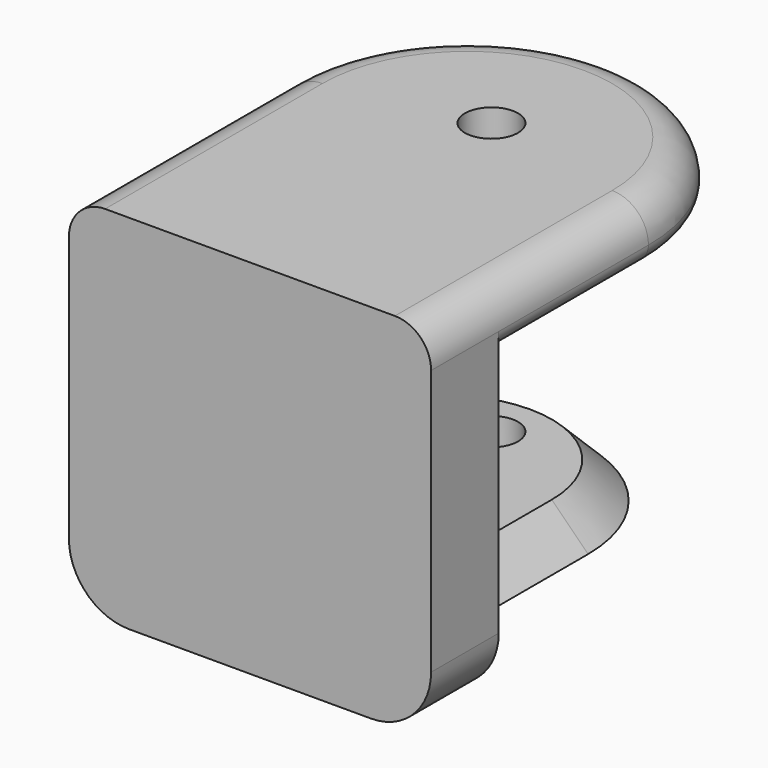
from build123d import *

# Parameters (mm, degrees)
F1_DEPTH  = 7
F3_DEPTH  = 4.5
F4_R      = 3
F5_R      = 1.49999
F7_D      = 4.4
F10_DEPTH = 3
F11_R     = 2.2
F12_DEPTH = 3
F13_SIZE  = 2.99999


# Not quite as in the source:
# - a fillet or chamfer is up to 0.001 mm smaller than in the source, because OpenCascade refuses the exact size


with BuildPart() as f1:
    # F0 (on Front) → F1 (new body)
    with BuildSketch(Plane.XZ):
        with BuildLine():
            Line((15, -10), (15, 15))
            Line((15, 15), (-15, 15))
            Line((-15, 15), (-15, -10))
            ThreePointArc((-15, -10), (-13.5355339059, -13.5355339059), (-10, -15))
            Line((-10, -15), (10, -15))
            ThreePointArc((10, -15), (13.5355339059, -13.5355339059), (15, -10))
        make_face()
    extrude(amount=F1_DEPTH)

    # F2 (on face) → F3 (join)
    with BuildSketch(Plane.XY.offset(15)):
        with BuildLine():
            Line((-15, 0), (-15, -7))
            Line((-15, -7), (15, -7))
            Line((15, -7), (15, 0))
            Line((15, 0), (15, 15.5))
            ThreePointArc((15, 15.5), (10.6066017178, 26.1066017178), (0, 30.5))
            ThreePointArc((0, 30.5), (-10.6066017178, 26.1066017178), (-15, 15.5))
            Line((-15, 15.5), (-15, 0))
        make_face()
    extrude(amount=-F3_DEPTH)

    # F4
    f4_edges = [f1.edges().sort_by_distance(p)[0] for p in [
        (15, 4.25, 15),
    ]]
    fillet(f4_edges, radius=F4_R)

    # F5 (radius 1.5 in the source; OpenCascade refuses exactly that, so slightly less here)
    f5_edges = [f1.edges().sort_by_distance(p)[0] for p in [
        (15, 7.75, 10.5),
    ]]
    fillet(f5_edges, radius=F5_R)

    # F7 (through all)
    with Locations(Plane.XY.offset(15)):
        with Locations((0, 18)):
            Hole(F7_D / 2)

    # F9 (on offset) → F10 (join)
    with BuildSketch(Plane(origin=(0, 0, -10.5), x_dir=(1, 0, 0), z_dir=(0, 0, -1))):
        with BuildLine():
            Line((12, 0), (-12, 0))
            Line((-12, 0), (-12, -13))
            ThreePointArc((-12, -13), (-8.4852813742, -21.4852813742), (0, -25))
            ThreePointArc((0, -25), (8.4852813742, -21.4852813742), (12, -13))
            Line((12, -13), (12, 0))
        make_face()
    extrude(amount=-F10_DEPTH)

    # F11 (on face) → F12 (cut)
    with BuildSketch(Plane(origin=(0, 0, -10.5), x_dir=(1, 0, 0), z_dir=(0, 0, -1))):
        with Locations((0, -18)):
            Circle(F11_R)
    extrude(amount=-F12_DEPTH, mode=Mode.SUBTRACT)

    # F13 (size 3 in the source; OpenCascade refuses exactly that, so slightly less here)
    f13_edges = [f1.edges().sort_by_distance(p)[0] for p in [
        (-12, 6.5, -7.5),
    ]]
    chamfer(f13_edges, length=F13_SIZE)


solid = f1.part
